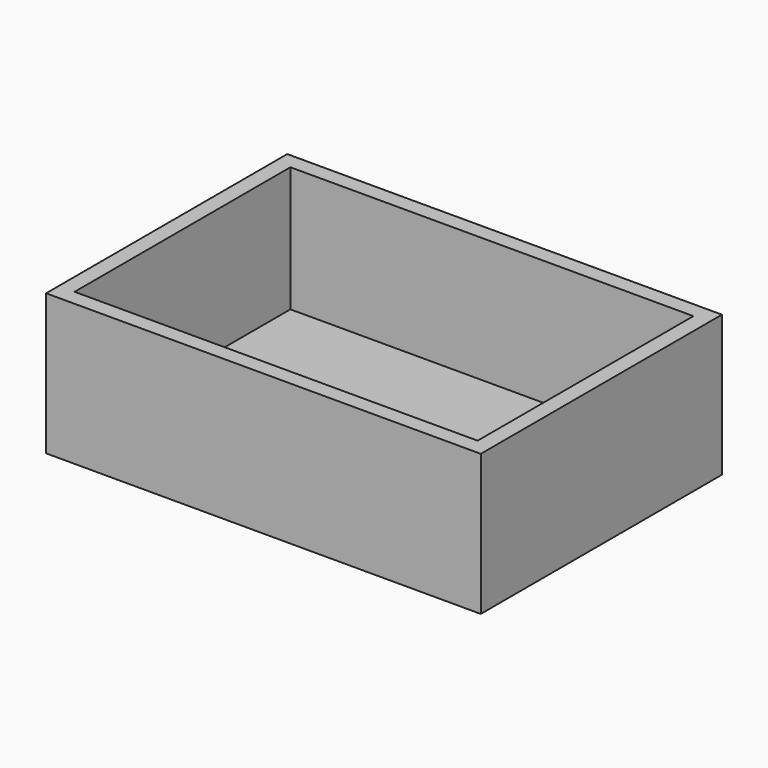
from build123d import *

# Parameters (mm, degrees)
F0_W     = 69.7228704538
F0_H     = 48.3472757041
F2_DEPTH = 22.606
F3_T     = -2.54


# Not quite as in the source:
# - the program builds the solid bodies; features that only make, move or delete a surface that nothing else refers to are left out


with BuildPart() as f2:
    # F0 (on Top) → F2 (new body)
    with BuildSketch(Plane.XY):
        with Locations((-0.3088367658, 0)):
            Rectangle(F0_W, F0_H)
    extrude(amount=F2_DEPTH)

    # F3
    f3_openings = [f2.faces().sort_by_distance(p)[0] for p in [
        (-0.308837, 0, 22.606),
    ]]
    offset(amount=F3_T, openings=f3_openings)


solid = f2.part
